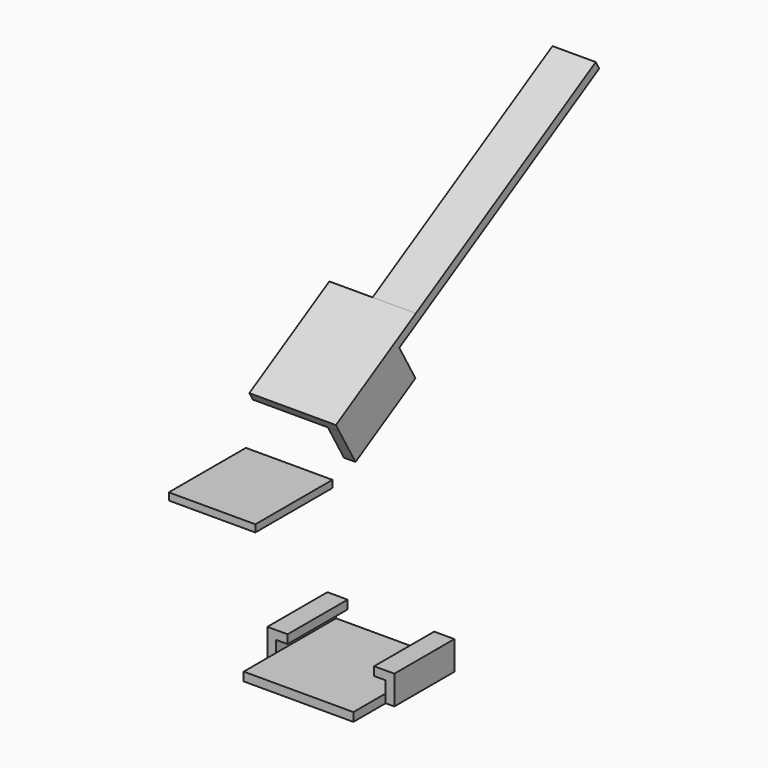
from build123d import *

# Parameters (mm, degrees)
F1_DEPTH  = 13
F0_W      = 19
F0_H      = 1.5
F2_DEPTH  = 20
F4_DEPTH  = 15
F6_W      = 7.5
F6_H      = 1.5
F7_DEPTH  = 45
F8_W      = 15.2
F8_H      = 1.25
F8_W_2    = 1.5
F9_DEPTH  = 15
F11_DEPTH = 2


# Not quite as in the source:
# - a feature names something its author has since deleted; it is built from what else it names


with BuildPart() as f1:
    # F0 (on Front) → F1 (new body)
    with BuildSketch(Plane.XZ):
        Polygon((-16.114479475, -31.1727552094), (-16.114479475, -29.6727552094), (-16.114479475, -27.6727552094), (-14.114479475, -27.6727552094), (-14.114479475, -26.1727552094), (-17.614479475, -26.1727552094), (-17.614479475, -31.1727552094), align=None)
    extrude(amount=F1_DEPTH)



with BuildPart() as f1b:
    # F0 (on Front) → F1, piece 2 (new body)
    with BuildSketch(Plane.XZ):
        Polygon((2.885520525, -27.6727552094), (2.885520525, -29.6727552094), (2.885520525, -31.1727552094), (4.385520525, -31.1727552094), (4.385520525, -26.1727552094), (0.885520525, -26.1727552094), (0.885520525, -27.6727552094), align=None)
    extrude(amount=F1_DEPTH)


with BuildPart() as f1_1:
    add(f1.part)

    add(f1b.part)  # F2 merges F1b
    # F0 (on Front) → F2 (join)
    with BuildSketch(Plane.XZ):
        with Locations((-6.614479475, -30.4227552094)):
            Rectangle(F0_W, F0_H)
    extrude(amount=F2_DEPTH)


with BuildPart() as f4:
    # F3 (on Right) → F4 (new body)
    with BuildSketch(Plane.YZ):
        Polygon((-21.6069256863, -37.1474194041), (-38.927433762, -47.1474194041), (-38.177433762, -48.4464575097), (-20.8569256863, -38.4464575097), align=None)
    extrude(amount=F4_DEPTH)


with BuildPart() as f4_1:
    # F5: moved
    add(f4.part.moved(Location((0, 0, 72.9))))

    # F6 (on face) → F7 (join)
    with BuildSketch(Plane(origin=(0, -0.7238727413, -0.417928122), x_dir=(-1, 0, 0), z_dir=(0, 0.8660254038, 0.5))):
        with Locations((-11.25, 41.0161058901)):
            Rectangle(F6_W, F6_H)
    extrude(amount=F7_DEPTH)

    # F10 (on face) → F11 (join)
    with BuildSketch(Plane.YZ.offset(15)):
        Polygon((-25.1870527052, 31.9535424903), (-38.177433762, 24.4535424903), (-34.677433762, 18.3913646638), (-21.6870527052, 25.8913646638), align=None)
    extrude(amount=-F11_DEPTH)


with BuildPart() as f9:
    # F8 (on face) → F9 (new body)
    with BuildSketch(Plane.YZ.offset(15)):
        with Locations((-47.277433762, 17.0785424903)):
            Rectangle(F8_W, F8_H)
        with Locations((-55.627433762, 17.0785424903)):
            Rectangle(F8_W_2, F8_H)
    extrude(amount=-F9_DEPTH)


solid = Compound([f1_1.part, f4_1.part, f9.part])
